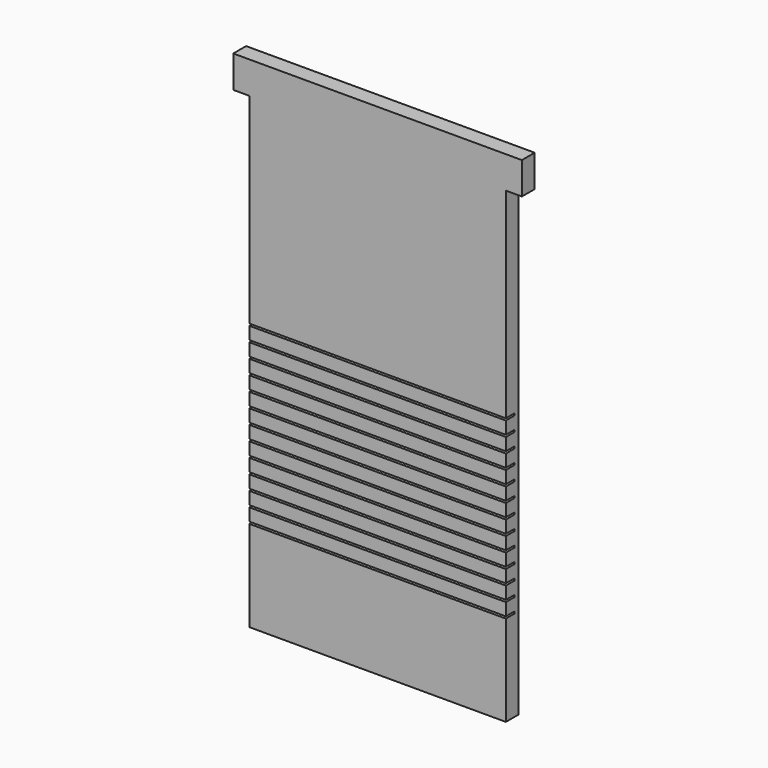
from build123d import *

# Parameters (mm, degrees)
F1_DEPTH = 25.4
F2_W     = 406.4
F2_H     = 3.175
F3_DEPTH = 17.4625


# Not quite as in the source:
# - a feature names something its author has since deleted; it is built from what else it names


with BuildPart() as f1:
    # F0 (on Front) → F1 (new body)
    with BuildSketch(Plane.XZ):
        Polygon((218.0226445198, -253.3499094963), (218.0226445198, 487.6006533037), (243.4226445198, 487.6006533037), (243.4226445198, 538.4006533037), (-213.7773554802, 538.4006533037), (-213.7773554802, 487.6006533037), (-188.3773554802, 487.6006533037), (-188.3773554802, -253.3499094963), align=None)
    extrude(amount=F1_DEPTH)

    # F2 (on face) → F3 (cut)
    with BuildSketch(Plane.XZ.offset(25.4)):
        with Locations((14.8226445198, 168.5131533037)):
            Rectangle(F2_W, F2_H)
        with Locations((14.8226445198, 145.4944033037)):
            Rectangle(F2_W, F2_H)
        with Locations((14.8226445198, 122.4756533037)):
            Rectangle(F2_W, F2_H)
        with Locations((14.8226445198, 7.3819033037)):
            Rectangle(F2_W, F2_H)
        with Locations((14.8226445198, 76.4381533037)):
            Rectangle(F2_W, F2_H)
        with Locations((14.8226445198, 53.4194033037)):
            Rectangle(F2_W, F2_H)
        with Locations((14.8226445198, 99.4569033037)):
            Rectangle(F2_W, F2_H)
        with Locations((14.8226445198, 30.4006533037)):
            Rectangle(F2_W, F2_H)
        with Locations((14.8226445198, -15.6368466963)):
            Rectangle(F2_W, F2_H)
        with Locations((14.8226445198, -38.6555966963)):
            Rectangle(F2_W, F2_H)
        with Locations((14.8226445198, -61.6743466963)):
            Rectangle(F2_W, F2_H)
        with Locations((14.8226445198, -84.6930966963)):
            Rectangle(F2_W, F2_H)
        with Locations((14.8226445198, -107.7118466963)):
            Rectangle(F2_W, F2_H)
    extrude(amount=-F3_DEPTH, mode=Mode.SUBTRACT)


solid = f1.part
